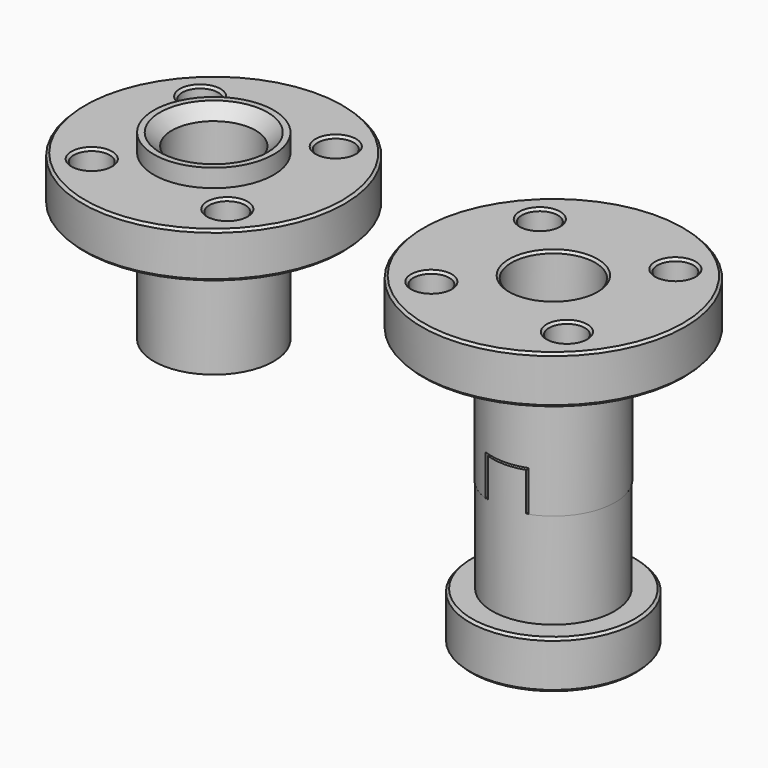
from build123d import *

# Parameters (mm, degrees)
F0_R       = 10.925
F0_R_2     = 1.5
F0_R_3     = 5
F1_DEPTH   = 3.8
F0_R_4     = 3.5
F2_DEPTH   = 5.3
F3_DEPTH   = 9.9
F4_SIZE    = 1
F5_SIZE    = 0.2
F0_R_5     = 11
F0_R_6     = 5.15
F6_DEPTH   = 4
F7_DEPTH   = 11
F9_R       = 5.1
F9_R_2     = 3.5
F10_DEPTH  = 15.2
F9_R_3     = 7
F11_DEPTH  = 4
F12_W      = 3.2
F12_H      = 3
F12_H_2    = 0.2
F12_W_2    = 0.2
F13_DEPTH  = 12.5
F12_W_3    = 3.35
F12_H_3    = 3.2
F14_DEPTH  = 12.5
F15_SIZE   = 0.2
F15_2_SIZE = 0.2


with BuildPart() as f1:
    # F0 (on Top) → F1 (new body)
    with BuildSketch(Plane.XY):
        with Locations((-28.3370425482, 7.17e-08)):
            Circle(F0_R)
        with Locations((-33.9938967977, -5.6568541778)):
            Circle(F0_R_2, mode=Mode.SUBTRACT)
        with Locations((-22.6801882987, -5.6568541778)):
            Circle(F0_R_2, mode=Mode.SUBTRACT)
        with Locations((-28.3370425482, 7.17e-08)):
            Circle(F0_R_3, mode=Mode.SUBTRACT)
        with Locations((-33.9938967977, 5.6568543212)):
            Circle(F0_R_2, mode=Mode.SUBTRACT)
        with Locations((-22.6801882987, 5.6568543212)):
            Circle(F0_R_2, mode=Mode.SUBTRACT)
    extrude(amount=F1_DEPTH)

    # F0 (on Top) → F2 (join)
    with BuildSketch(Plane.XY):
        with Locations((-28.3370425482, 7.17e-08)):
            Circle(F0_R_3)
        with Locations((-28.3370425482, 7.17e-08)):
            Circle(F0_R_4, mode=Mode.SUBTRACT)
    extrude(amount=F2_DEPTH)

    # F0 (on Top) → F3 (join)
    with BuildSketch(Plane.XY):
        with Locations((-28.3370425482, 7.17e-08)):
            Circle(F0_R_3)
        with Locations((-28.3370425482, 7.17e-08)):
            Circle(F0_R_4, mode=Mode.SUBTRACT)
    extrude(amount=-F3_DEPTH)

    # F4
    f4_edges = [f1.edges().sort_by_distance(p)[0] for p in [
        (-31.837043, 0, 5.3),
        (-31.837043, 0, -9.9),
    ]]
    chamfer(f4_edges, length=F4_SIZE)

    # F5
    f5_edges = [f1.edges().sort_by_distance(p)[0] for p in [
        (-35.493897, 5.656854, 3.8),
        (-35.493897, -5.656854, 3.8),
        (-24.180188, -5.656854, 3.8),
        (-24.180188, 5.656854, 3.8),
        (-39.262043, 0, 3.8),
        (-39.262043, 0, 0),
    ]]
    chamfer(f5_edges, length=F5_SIZE)


with BuildPart() as f6:
    # F0 (on Top) → F6 (new body)
    with BuildSketch(Plane.XY):
        Circle(F0_R_5)
        with Locations((-5.6568542495, -5.6568542495)):
            Circle(F0_R_2, mode=Mode.SUBTRACT)
        with Locations((5.6568542495, -5.6568542495)):
            Circle(F0_R_2, mode=Mode.SUBTRACT)
        Circle(F0_R_6, mode=Mode.SUBTRACT)
        with Locations((-5.6568542495, 5.6568542495)):
            Circle(F0_R_2, mode=Mode.SUBTRACT)
        with Locations((5.6568542495, 5.6568542495)):
            Circle(F0_R_2, mode=Mode.SUBTRACT)
        Circle(F0_R_6)
        Circle(F0_R_4, mode=Mode.SUBTRACT)
    extrude(amount=F6_DEPTH)

    # F0 (on Top) → F7 (join)
    with BuildSketch(Plane.XY):
        Circle(F0_R_6)
        Circle(F0_R_4, mode=Mode.SUBTRACT)
    extrude(amount=-F7_DEPTH)

    # F12 (on Front) → F13 (cut, symmetric)
    with BuildSketch(Plane.XZ):
        with Locations((0, -9.3)):
            Rectangle(F12_W, F12_H)
        with Locations((0, -10.9)):
            Rectangle(F12_W, F12_H_2)
        with Locations((-1.7, -10.9)):
            Rectangle(F12_W_2, F12_H_2)
        Polygon((-1.8, -7.6), (-1.8, -10.8), (-1.6, -10.8), (-1.6, -7.8), (1.6, -7.8), (1.6, -10.8), (1.8, -10.8), (1.8, -7.6), align=None)
        with Locations((1.7, -10.9)):
            Rectangle(F12_W_2, F12_H_2)
    extrude(amount=F13_DEPTH, both=True, mode=Mode.SUBTRACT)

    # F15
    f15_edges = [f6.edges().sort_by_distance(p)[0] for p in [
        (-3.5, 0, 4),
        (-11, 0, 4),
        (-7.156854, -5.656854, 4),
        (4.156854, -5.656854, 4),
        (4.156854, 5.656854, 4),
        (-7.156854, 5.656854, 4),
        (-11, 0, 0),
    ]]
    chamfer(f15_edges, length=F15_SIZE)


with BuildPart() as f10:
    # F9 (on offset) → F10 (new body)
    with BuildSketch(Plane(origin=(0, 0, -23), x_dir=(1, 0, 0), z_dir=(0, 0, -1))):
        Circle(F9_R)
        Circle(F9_R_2, mode=Mode.SUBTRACT)
    extrude(amount=-F10_DEPTH)

    # F9 (on offset) → F11 (join)
    with BuildSketch(Plane(origin=(0, 0, -23), x_dir=(1, 0, 0), z_dir=(0, 0, -1))):
        Circle(F9_R_3)
        Circle(F9_R, mode=Mode.SUBTRACT)
    extrude(amount=-F11_DEPTH)

    # F12 (on Front) → F14 (cut, symmetric)
    with BuildSketch(Plane.XZ):
        Polygon((-1.8, -7.6), (-1.8, -10.8), (-1.6, -10.8), (-1.6, -7.8), (1.6, -7.8), (1.6, -10.8), (1.8, -10.8), (1.8, -7.6), align=None)
        with Locations((-3.475, -9.2)):
            Rectangle(F12_W_3, F12_H_3)
        with Locations((3.475, -9.2)):
            Rectangle(F12_W_3, F12_H_3)
        with Locations((-3.475, -10.9)):
            Rectangle(F12_W_3, F12_H_2)
        with Locations((-1.7, -10.9)):
            Rectangle(F12_W_2, F12_H_2)
        with Locations((1.7, -10.9)):
            Rectangle(F12_W_2, F12_H_2)
        with Locations((3.475, -10.9)):
            Rectangle(F12_W_3, F12_H_2)
    extrude(amount=F14_DEPTH, both=True, mode=Mode.SUBTRACT)

    # F15#2
    f15_2_edges = [f10.edges().sort_by_distance(p)[0] for p in [
        (-7, 0, -19),
        (-7, 0, -23),
    ]]
    chamfer(f15_2_edges, length=F15_2_SIZE)


solid = Compound([f1.part, f6.part, f10.part])
